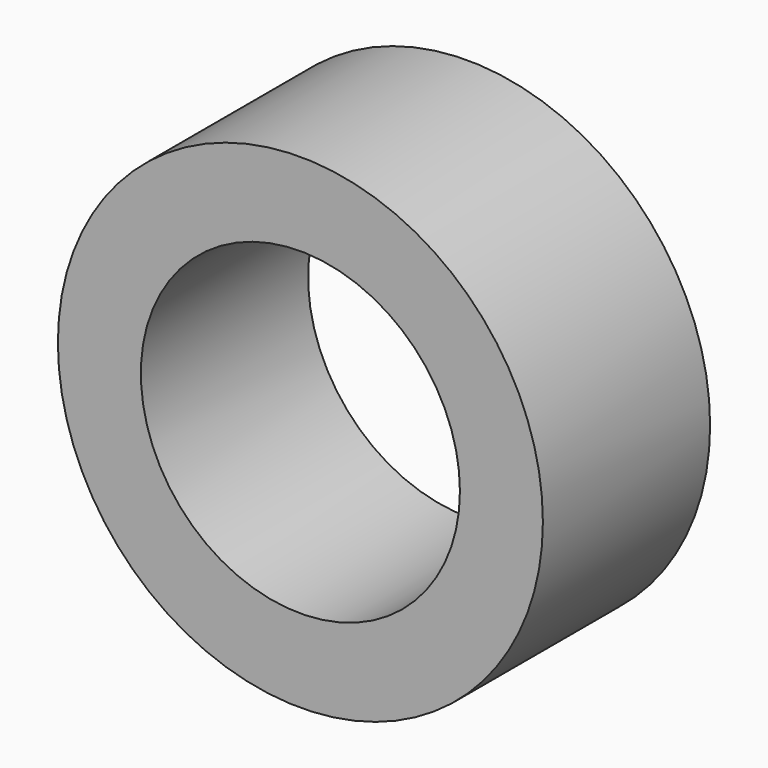
from build123d import *

# Parameters (mm, degrees)
F0_R     = 17.6806314322
F1_DEPTH = 15.24
F3_R     = 11.6315842242
F4_DEPTH = 15.24


# Not quite as in the source:
# - the program builds the solid bodies; features that only make, move or delete a surface that nothing else refers to are left out


with BuildPart() as f1:
    # F0 (on Front) → F1 (new body)
    with BuildSketch(Plane.XZ):
        with Locations((0, 51.8556125462)):
            Circle(F0_R)
    extrude(amount=F1_DEPTH)

    # F3 (on face) → F4 (cut)
    with BuildSketch(Plane.XZ.offset(15.24)):
        with Locations((0, 51.8556125462)):
            Circle(F3_R)
    extrude(amount=-F4_DEPTH, mode=Mode.SUBTRACT)


solid = f1.part
